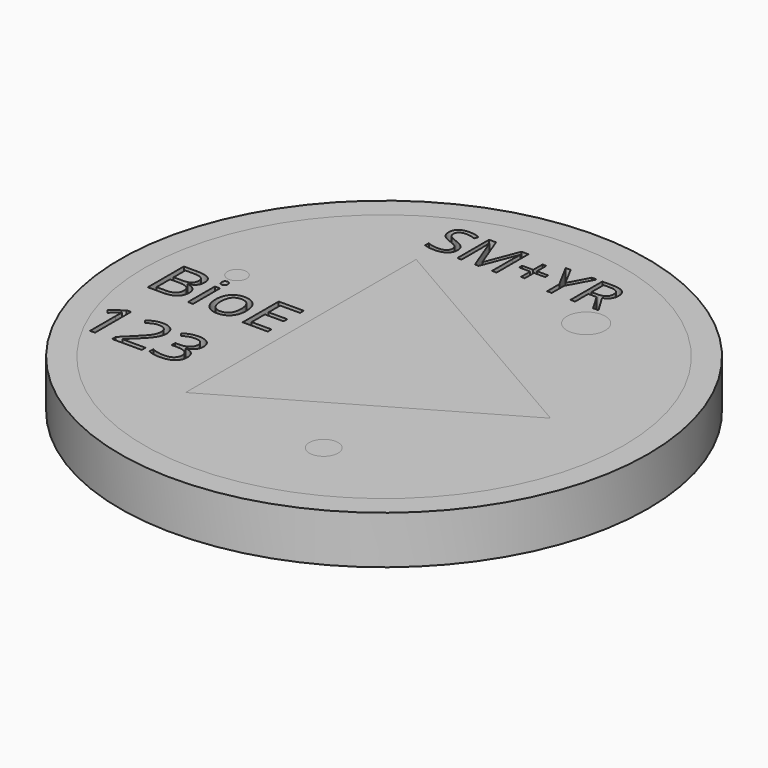
from build123d import *

# Parameters (mm, degrees)
F0_R           = 27.5
F1_DEPTH       = 5
F2_R           = 25
F2_R_2         = 1.5
F2_R_3         = 1
F2_R_4         = 2
F3_DEPTH       = 3
F4_DEPTH       = 3
F5_DEPTH       = 3
F6_TEXT_SIZE   = 5.7966344886
F6_TEXT_SIZE_2 = 6.5688326787
F7_DEPTH       = 1
F8_DEPTH       = 1.5


# Not quite as in the source:
# - Text() gives the source's letters only with a copy of the font that has no kerning and outlines rounded to 1/6400 em; it was checked with that copy


with BuildPart() as f1:
    # F0 (on Top) → F1 (new body)
    with BuildSketch(Plane.XY):
        Circle(F0_R)
    extrude(amount=F1_DEPTH)

    # F2 (on face) → F3 (cut)
    with BuildSketch(Plane.XY.offset(5)):
        Circle(F2_R)
        with Locations((6.1927237548, -15.6056657434)):
            Circle(F2_R_2, mode=Mode.SUBTRACT)
        with Locations((-18.3304660022, 3.7578297779)):
            Circle(F2_R_3, mode=Mode.SUBTRACT)
        Polygon((17.3396281898, 0), (-8.6698140949, -15.0165585045), (-8.6698140949, 15.0165585045), align=None, mode=Mode.SUBTRACT)
        with Locations((9.1652339324, 14.8625392467)):
            Circle(F2_R_4, mode=Mode.SUBTRACT)
    extrude(amount=-F3_DEPTH, mode=Mode.SUBTRACT)

    # F2 (on face) → F4 (join)
    with BuildSketch(Plane.XY.offset(5)):
        Polygon((-8.6698140949, 15.0165585045), (-8.6698140949, -15.0165585045), (17.3396281898, 0), align=None)
    extrude(amount=-F4_DEPTH)


with BuildPart() as f5:
    # F5 (new): a face of the model
    f5_faces = [f1.part.faces().sort_by_distance(p)[0] for p in [
        (-24.2928932188, 0, 2),
    ]]
    extrude(f5_faces, amount=F5_DEPTH)

    # F6 (on face) → F7 (cut)
    with BuildSketch(Plane.XY.offset(5)):
        with Locations((-9.9570071325, 17.2934513539)):
            Text('SM+YR', F6_TEXT_SIZE, font='Open Sans', text_align=(TextAlign.LEFT, TextAlign.BOTTOM))
        with Locations((-23.3015343547, -2.4507237831)):
            Text('BioE', F6_TEXT_SIZE_2, font='Open Sans', text_align=(TextAlign.LEFT, TextAlign.BOTTOM))
        with Locations((-23.3015343547, -11.3843362261)):
            Text('123', F6_TEXT_SIZE_2, font='Open Sans', text_align=(TextAlign.LEFT, TextAlign.BOTTOM))
    extrude(amount=-F7_DEPTH, mode=Mode.SUBTRACT)

    # F6 (on face) → F8 (cut)
    with BuildSketch(Plane.XY.offset(5)):
        with Locations((-9.9570071325, 17.2934513539)):
            Text('SM+YR', F6_TEXT_SIZE, font='Open Sans', text_align=(TextAlign.LEFT, TextAlign.BOTTOM))
        with Locations((-23.3015343547, -2.4507237831)):
            Text('BioE', F6_TEXT_SIZE_2, font='Open Sans', text_align=(TextAlign.LEFT, TextAlign.BOTTOM))
        with Locations((-23.3015343547, -11.3843362261)):
            Text('123', F6_TEXT_SIZE_2, font='Open Sans', text_align=(TextAlign.LEFT, TextAlign.BOTTOM))
    extrude(amount=-F8_DEPTH, mode=Mode.SUBTRACT)


solid = Compound([f1.part, f5.part])
